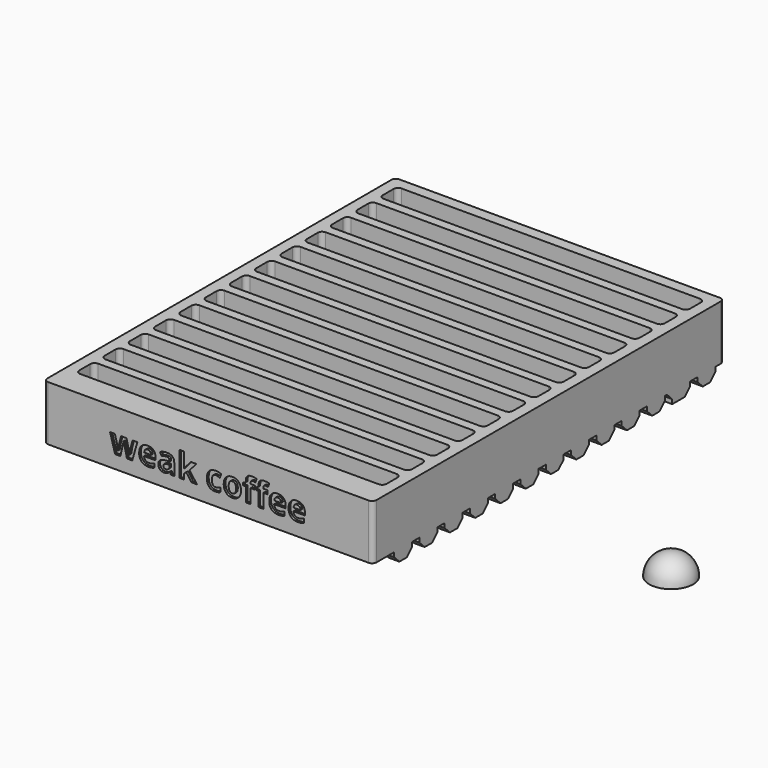
from build123d import *

# Parameters (mm, degrees)
F0_W         = 150
F0_H         = 200
F0_W_2       = 140
F0_H_2       = 10.2
F1_DEPTH     = 25
F2_W         = 5
F2_H         = 10.2
F3_DEPTH     = 5
F4_SIZE      = 3
F7_R         = 2
F8_TEXT_SIZE = 14.8809534342
F9_DEPTH     = 1
F11_ANGLE    = 180


# Not quite as in the source:
# - Text() gives the source's letters only with a copy of the font that has no kerning and outlines rounded to 1/6400 em; it was checked with that copy


with BuildPart() as f1:
    # F0 (on Top) → F1 (new body)
    with BuildSketch(Plane.XY):
        with Locations((-25.513516739, 120.3928657384)):
            Rectangle(F0_W, F0_H)
        with Locations((-25.513516739, 37.4928657384)):
            Rectangle(F0_W_2, F0_H_2, mode=Mode.SUBTRACT)
        with Locations((-25.513516739, 51.8928657384)):
            Rectangle(F0_W_2, F0_H_2, mode=Mode.SUBTRACT)
        with Locations((-25.513516739, 66.2928657384)):
            Rectangle(F0_W_2, F0_H_2, mode=Mode.SUBTRACT)
        with Locations((-25.513516739, 80.6928657384)):
            Rectangle(F0_W_2, F0_H_2, mode=Mode.SUBTRACT)
        with Locations((-25.513516739, 95.0928657384)):
            Rectangle(F0_W_2, F0_H_2, mode=Mode.SUBTRACT)
        with Locations((-25.513516739, 109.4928657384)):
            Rectangle(F0_W_2, F0_H_2, mode=Mode.SUBTRACT)
        with Locations((-25.513516739, 123.8928657384)):
            Rectangle(F0_W_2, F0_H_2, mode=Mode.SUBTRACT)
        with Locations((-25.513516739, 138.2928657384)):
            Rectangle(F0_W_2, F0_H_2, mode=Mode.SUBTRACT)
        with Locations((-25.513516739, 152.6928657384)):
            Rectangle(F0_W_2, F0_H_2, mode=Mode.SUBTRACT)
        with Locations((-25.513516739, 167.0928657384)):
            Rectangle(F0_W_2, F0_H_2, mode=Mode.SUBTRACT)
        with Locations((-25.513516739, 181.4928657384)):
            Rectangle(F0_W_2, F0_H_2, mode=Mode.SUBTRACT)
        with Locations((-25.513516739, 195.8928657384)):
            Rectangle(F0_W_2, F0_H_2, mode=Mode.SUBTRACT)
        with Locations((-25.513516739, 210.2928657384)):
            Rectangle(F0_W_2, F0_H_2, mode=Mode.SUBTRACT)
    extrude(amount=F1_DEPTH)

    # F2 (on face) → F3 (join)
    with BuildSketch(Plane(origin=(0, 0, 0), x_dir=(1, 0, 0), z_dir=(0, 0, -1))):
        with Locations((-98.013516739, -210.2928657384)):
            Rectangle(F2_W, F2_H)
        with Locations((-98.013516739, -195.8928657384)):
            Rectangle(F2_W, F2_H)
        with Locations((-98.013516739, -181.4928657384)):
            Rectangle(F2_W, F2_H)
        with Locations((-98.013516739, -167.0928657384)):
            Rectangle(F2_W, F2_H)
        with Locations((-98.013516739, -152.6928657384)):
            Rectangle(F2_W, F2_H)
        with Locations((-98.013516739, -138.2928657384)):
            Rectangle(F2_W, F2_H)
        with Locations((-98.013516739, -123.8928657384)):
            Rectangle(F2_W, F2_H)
        with Locations((-98.013516739, -109.4928657384)):
            Rectangle(F2_W, F2_H)
        with Locations((-98.013516739, -95.0928657384)):
            Rectangle(F2_W, F2_H)
        with Locations((-98.013516739, -80.6928657384)):
            Rectangle(F2_W, F2_H)
        with Locations((-98.013516739, -66.2928657384)):
            Rectangle(F2_W, F2_H)
        with Locations((-98.013516739, -51.8928657384)):
            Rectangle(F2_W, F2_H)
        with Locations((-98.013516739, -37.4928657384)):
            Rectangle(F2_W, F2_H)
        with Locations((46.986483261, -210.2928657384)):
            Rectangle(F2_W, F2_H)
        with Locations((46.986483261, -195.8928657384)):
            Rectangle(F2_W, F2_H)
        with Locations((46.986483261, -181.4928657384)):
            Rectangle(F2_W, F2_H)
        with Locations((46.986483261, -167.0928657384)):
            Rectangle(F2_W, F2_H)
        with Locations((46.986483261, -152.6928657384)):
            Rectangle(F2_W, F2_H)
        with Locations((46.986483261, -138.2928657384)):
            Rectangle(F2_W, F2_H)
        with Locations((46.986483261, -123.8928657384)):
            Rectangle(F2_W, F2_H)
        with Locations((46.986483261, -109.4928657384)):
            Rectangle(F2_W, F2_H)
        with Locations((46.986483261, -95.0928657384)):
            Rectangle(F2_W, F2_H)
        with Locations((46.986483261, -80.6928657384)):
            Rectangle(F2_W, F2_H)
        with Locations((46.986483261, -66.2928657384)):
            Rectangle(F2_W, F2_H)
        with Locations((46.986483261, -51.8928657384)):
            Rectangle(F2_W, F2_H)
        with Locations((46.986483261, -37.4928657384)):
            Rectangle(F2_W, F2_H)
    extrude(amount=F3_DEPTH)

    # F4
    f4_edges = [f1.edges().sort_by_distance(p)[0] for p in [
        (-98.013517, 215.392866, -5),
        (-98.013517, 205.192866, -5),
        (-98.013517, 200.992866, -5),
        (-98.013517, 190.792866, -5),
        (-98.013517, 186.592866, -5),
        (-98.013517, 176.392866, -5),
        (-98.013517, 172.192866, -5),
        (-98.013517, 161.992866, -5),
        (-98.013517, 157.792866, -5),
        (-98.013517, 147.592866, -5),
        (-98.013517, 143.392866, -5),
        (-98.013517, 133.192866, -5),
        (-98.013517, 128.992866, -5),
        (-98.013517, 118.792866, -5),
        (-98.013517, 114.592866, -5),
        (-98.013517, 104.392866, -5),
        (-98.013517, 100.192866, -5),
        (-98.013517, 89.992866, -5),
        (-98.013517, 85.792866, -5),
        (-98.013517, 75.592866, -5),
        (-98.013517, 71.392866, -5),
        (-98.013517, 61.192866, -5),
        (-98.013517, 56.992866, -5),
        (-98.013517, 46.792866, -5),
        (-98.013517, 42.592866, -5),
        (-98.013517, 32.392866, -5),
        (46.986483, 32.392866, -5),
        (46.986483, 42.592866, -5),
        (46.986483, 56.992866, -5),
        (46.986483, 46.792866, -5),
        (46.986483, 71.392866, -5),
        (46.986483, 61.192866, -5),
        (46.986483, 75.592866, -5),
        (46.986483, 85.792866, -5),
        (46.986483, 89.992866, -5),
        (46.986483, 100.192866, -5),
        (46.986483, 104.392866, -5),
        (46.986483, 114.592866, -5),
        (46.986483, 118.792866, -5),
        (46.986483, 128.992866, -5),
        (46.986483, 133.192866, -5),
        (46.986483, 143.392866, -5),
        (46.986483, 147.592866, -5),
        (46.986483, 157.792866, -5),
        (46.986483, 161.992866, -5),
        (46.986483, 172.192866, -5),
        (46.986483, 176.392866, -5),
        (46.986483, 186.592866, -5),
        (46.986483, 190.792866, 0),
        (46.986483, 200.992866, -5),
        (46.986483, 205.192866, -5),
        (46.986483, 215.392866, -5),
    ]]
    chamfer(f4_edges, length=F4_SIZE)

    # F5 (on face) → F6 (revolve, cut)
    with BuildSketch(Plane(origin=(0, 0, 0), x_dir=(1, 0, 0), z_dir=(0, 0, -1))):
        with BuildLine():
            Line((-1.013516739, -109.4928657384), (19.986483261, -109.4928657384))
            ThreePointArc((19.986483261, -109.4928657384), (9.486483261, -98.9928657384), (-1.013516739, -109.4928657384))
        make_face()
        with BuildLine():
            Line((-71.013516739, -109.4928657384), (-50.013516739, -109.4928657384))
            ThreePointArc((-50.013516739, -109.4928657384), (-60.513516739, -98.9928657384), (-71.013516739, -109.4928657384))
        make_face()
    revolve(axis=Axis((-60.513516739, 109.4928657384, 0), (1, 0, 0)), mode=Mode.SUBTRACT)

    # F7
    f7_edges = [f1.edges().sort_by_distance(p)[0] for p in [
        (-100.513517, 20.392866, 12.5),
        (49.486483, 20.392866, 12.5),
        (49.486483, 220.392866, 12.5),
        (-100.513517, 220.392866, 12.5),
        (44.486483, 176.392866, 12.5),
        (44.486483, 190.792866, 12.5),
        (44.486483, 205.192866, 12.5),
        (44.486483, 161.992866, 12.5),
        (44.486483, 147.592866, 12.5),
        (44.486483, 133.192866, 12.5),
        (44.486483, 118.792866, 12.5),
        (44.486483, 104.392866, 12.5),
        (44.486483, 89.992866, 12.5),
        (44.486483, 75.592866, 12.5),
        (44.486483, 61.192866, 12.5),
        (44.486483, 46.792866, 12.5),
        (44.486483, 32.392866, 12.5),
        (44.486483, 215.392866, 12.5),
        (44.486483, 200.992866, 12.5),
        (44.486483, 186.592866, 12.5),
        (44.486483, 172.192866, 12.5),
        (44.486483, 157.792866, 12.5),
        (44.486483, 143.392866, 12.5),
        (44.486483, 128.992866, 12.5),
        (44.486483, 114.592866, 12.5),
        (44.486483, 100.192866, 12.5),
        (44.486483, 85.792866, 12.5),
        (44.486483, 71.392866, 12.5),
        (44.486483, 56.992866, 12.5),
        (44.486483, 42.592866, 12.5),
        (-95.513517, 205.192866, 12.5),
        (-95.513517, 190.792866, 12.5),
        (-95.513517, 176.392866, 12.5),
        (-95.513517, 161.992866, 12.5),
        (-95.513517, 147.592866, 12.5),
        (-95.513517, 133.192866, 12.5),
        (-95.513517, 118.792866, 12.5),
        (-95.513517, 104.392866, 12.5),
        (-95.513517, 89.992866, 12.5),
        (-95.513517, 75.592866, 12.5),
        (-95.513517, 61.192866, 12.5),
        (-95.513517, 46.792866, 12.5),
        (-95.513517, 32.392866, 12.5),
        (-95.513517, 215.392866, 12.5),
        (-95.513517, 200.992866, 12.5),
        (-95.513517, 186.592866, 12.5),
        (-95.513517, 172.192866, 12.5),
        (-95.513517, 157.792866, 12.5),
        (-95.513517, 143.392866, 12.5),
        (-95.513517, 128.992866, 12.5),
        (-95.513517, 114.592866, 12.5),
        (-95.513517, 100.192866, 12.5),
        (-95.513517, 85.792866, 12.5),
        (-95.513517, 71.392866, 12.5),
        (-95.513517, 56.992866, 12.5),
        (-95.513517, 42.592866, 12.5),
    ]]
    fillet(f7_edges, radius=F7_R)

    # F8 (on face) → F9 (cut)
    with BuildSketch(Plane.XZ.offset(-20.3928657384)):
        with Locations((-70.4691095787, 6)):
            Text('weak coffee', F8_TEXT_SIZE, font='Open Sans', font_style=FontStyle.BOLD, text_align=(TextAlign.LEFT, TextAlign.BOTTOM))
    extrude(amount=-F9_DEPTH, mode=Mode.SUBTRACT)


with BuildPart() as f11:
    # F10 (on Top) → F11 (revolve)
    with BuildSketch(Plane.XY):
        with BuildLine():
            Line((128.0092352629, 79.5398131013), (148.0092352629, 79.5398131013))
            ThreePointArc((148.0092352629, 79.5398131013), (138.0092352629, 89.5398131013), (128.0092352629, 79.5398131013))
        make_face()
    revolve(axis=Axis((138.0092352629, 79.5398131013, 0), (1, 0, 0)), revolution_arc=F11_ANGLE)


solid = Compound([f1.part, f11.part])
